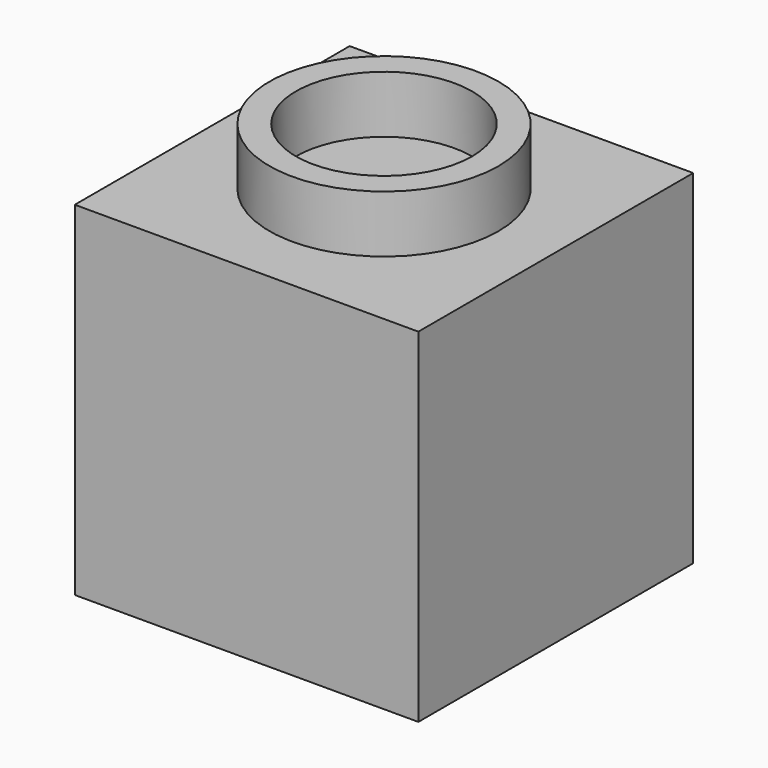
from build123d import *

# Parameters (mm, degrees)
F0_W     = 60
F0_H     = 60
F1_DEPTH = 30
F2_DEPTH = 30
F3_R     = 20
F4_DEPTH = 10
F6_R     = 15.3845355262
F7_DEPTH = 10
F8_W     = 60
F8_H     = 60
F9_DEPTH = 4


with BuildPart() as f1:
    # F0 (on Top) → F1 (new body)
    with BuildSketch(Plane.XY):
        Rectangle(F0_W, F0_H)
    extrude(amount=F1_DEPTH)

    # F2 (add): a face of the model
    f2_faces = [f1.faces().sort_by_distance(p)[0] for p in [
        (0, 0, 0),
    ]]
    extrude(f2_faces, amount=F2_DEPTH)

    # F3 (on face) → F4 (join)
    with BuildSketch(Plane.XY.offset(30)):
        Circle(F3_R)
    extrude(amount=F4_DEPTH)

    # F6 (on face) → F7 (cut)
    with BuildSketch(Plane.XY.offset(40)):
        Circle(F6_R)
    extrude(amount=-F7_DEPTH, mode=Mode.SUBTRACT)

    # F8 (on face) → F9 (cut)
    with BuildSketch(Plane(origin=(0, 30, 0), x_dir=(-1, 0, 0), z_dir=(0, 1, 0))):
        Rectangle(F8_W, F8_H)
    extrude(amount=F9_DEPTH, mode=Mode.SUBTRACT)


solid = f1.part
